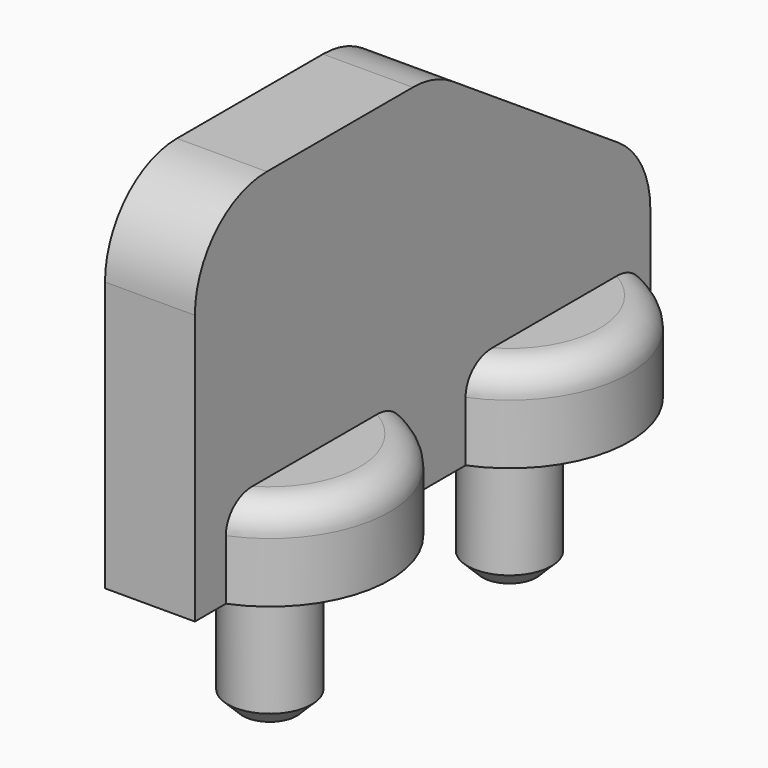
from build123d import *

# Parameters (mm, degrees)
F0_R     = 1.4
F1_DEPTH = 12
F2_DEPTH = 5
F3_SIZE  = 0.5
F4_DEPTH = 3
F5_R     = 1
F7_DEPTH = 25
F8_R     = 3


# Not quite as in the source:
# - a pattern or mirror of a feature is missing from the dataset's text; its kind, count and spacing are read off the source's solid
# - a feature names something its author has since deleted; it is built from what else it names


with BuildPart() as f1:
    # F0 (on Top) → F1 (new body)
    with BuildSketch(Plane.XY):
        with BuildLine():
            ThreePointArc((1.5, 8.7080992435), (0.7640690498, 8.92634671), (0, 9))
            ThreePointArc((0, 9), (-0.7640690498, 8.92634671), (-1.5, 8.7080992435))
            Line((-1.5, 8.7080992435), (-1.5, 1.2919007565))
            Line((-1.5, 1.2919007565), (-1.5, -1.2919007565))
            Line((-1.5, -1.2919007565), (-1.5, -8.7080992435))
            Line((-1.5, -8.7080992435), (-1.5, -10))
            Line((-1.5, -10), (1.5, -10))
            Line((1.5, -10), (1.5, -8.7080992435))
            Line((1.5, -8.7080992435), (1.5, -1.2919007565))
            Line((1.5, -1.2919007565), (1.5, 1.2919007565))
            Line((1.5, 1.2919007565), (1.5, 8.7080992435))
        make_face()
        with Locations((0, -5)):
            Circle(F0_R, mode=Mode.SUBTRACT)
        with Locations((0, 5)):
            Circle(F0_R, mode=Mode.SUBTRACT)
        with Locations((0, 5)):
            Circle(F0_R)
        with Locations((0, -5)):
            Circle(F0_R)
        with BuildLine():
            Line((0, 9), (-1.5, 9))
            Line((-1.5, 9), (-1.5, 8.7080992435))
            ThreePointArc((-1.5, 8.7080992435), (-0.7640690498, 8.92634671), (0, 9))
        make_face()
        with BuildLine():
            Line((1.5, 9), (0, 9))
            ThreePointArc((0, 9), (0.7640690498, 8.92634671), (1.5, 8.7080992435))
            Line((1.5, 8.7080992435), (1.5, 9))
        make_face()
    extrude(amount=F1_DEPTH)

    # F0 (on Top) → F2 (join)
    with BuildSketch(Plane.XY):
        with Locations((0, 5)):
            Circle(F0_R)
    f2 = extrude(amount=-F2_DEPTH)

    # F2_copies: F2 across plane
    add(f2.mirror(Plane(origin=(0, 0, 0), x_dir=(0, 0, -1), z_dir=(0, -1, 0))))

    # F3
    f3_edges = [f1.edges().sort_by_distance(p)[0] for p in [
        (-1.4, -5, -5),
        (-1.4, 5, -5),
    ]]
    chamfer(f3_edges, length=F3_SIZE)

    # F0 (on Top) → F4 (join)
    with BuildSketch(Plane.XY):
        with Locations((0, 5)):
            Circle(F0_R)
        with Locations((0, -5)):
            Circle(F0_R)
        with BuildLine():
            Line((0, 9), (-1.5, 9))
            Line((-1.5, 9), (-1.5, 8.7080992435))
            ThreePointArc((-1.5, 8.7080992435), (-0.7640690498, 8.92634671), (0, 9))
        make_face()
        with BuildLine():
            Line((1.5, 9), (0, 9))
            ThreePointArc((0, 9), (0.7640690498, 8.92634671), (1.5, 8.7080992435))
            Line((1.5, 8.7080992435), (1.5, 9))
        make_face()
        with BuildLine():
            Line((-1.5, 1.2919007565), (-1.5, 8.7080992435))
            ThreePointArc((-1.5, 8.7080992435), (-4, 5), (-1.5, 1.2919007565))
        make_face()
        with BuildLine():
            ThreePointArc((1.5, 1.2919007565), (4, 5), (1.5, 8.7080992435))
            Line((1.5, 8.7080992435), (1.5, 1.2919007565))
        make_face()
        with BuildLine():
            Line((-1.5, -8.7080992435), (-1.5, -1.2919007565))
            ThreePointArc((-1.5, -1.2919007565), (-4, -5), (-1.5, -8.7080992435))
        make_face()
        with BuildLine():
            ThreePointArc((1.5, -8.7080992435), (4, -5), (1.5, -1.2919007565))
            Line((1.5, -1.2919007565), (1.5, -8.7080992435))
        make_face()
    extrude(amount=F4_DEPTH)

    # F5
    f5_edges = [f1.edges().sort_by_distance(p)[0] for p in [
        (-4, -5, 3),
        (4, -5, 3),
        (-4, 5, 3),
        (4, 5, 3),
    ]]
    fillet(f5_edges, radius=F5_R)

    # F6 (on face) → F7 (cut)
    with BuildSketch(Plane(origin=(-1.5, 0, 0), x_dir=(0, -1, 0), z_dir=(-1, 0, 0))):
        Polygon((0, 12), (-9, 12), (-9, 6), align=None)
    extrude(amount=-F7_DEPTH, mode=Mode.SUBTRACT)

    # F8
    f8_edges = [f1.edges().sort_by_distance(p)[0] for p in [
        (0, -10, 12),
        (0, 0, 12),
        (0, 9, 6),
    ]]
    fillet(f8_edges, radius=F8_R)


solid = f1.part
